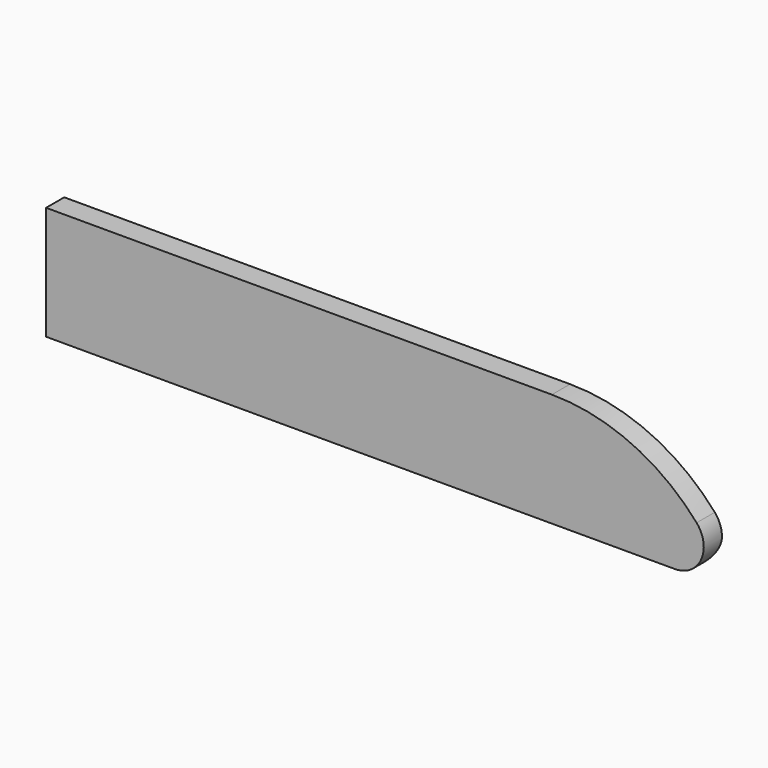
from build123d import *

# Parameters (mm, degrees)
F0_W        = 900
F0_H        = 150
F1_DEPTH    = 30
F2_T1_DEPTH = 1188.6630226256
F3_T1_DEPTH = 405.2304260538
F3_T3_DEPTH = 1086.1451046899


# Not quite as in the source:
# - a fillet or chamfer that OpenCascade refuses, or shapes differently, is made with other operations: its cross-section is extruded or revolved along the edge and cut away or added


with BuildPart() as f1:
    # F0 (on Front) → F1 (new body)
    with BuildSketch(Plane.XZ):
        with Locations((-450, -75)):
            Rectangle(F0_W, F0_H)
    extrude(amount=F1_DEPTH)

    # F2: fillet of radius 254 on 1 edges, made by hand

    # F2_s2 → F2_t1 (cut)
    with BuildSketch(Plane.XZ.offset(-579.3315113128)):
        with BuildLine():
            ThreePointArc((0, -150), (-93.7108671067, -40.7724220463), (-231.7326045251, 0))
            Line((-231.7326045251, 0), (0, 0))
            Line((0, 0), (0, -150))
        make_face()
    extrude(amount=F2_T1_DEPTH, mode=Mode.SUBTRACT)

    # F3: fillet of radius 38.1 on 2 edges, made by hand

    # F3_s2 → F3_t1 (cut)
    with BuildSketch(Plane.XZ.offset(-187.6152130269)):
        with BuildLine():
            ThreePointArc((-69.1890718946, -150), (-34.4974048158, -127.6511344129), (-40.5049190775, -86.8235294118))
            ThreePointArc((-40.5049190775, -86.8235294118), (-17.9063471748, -116.9075798319), (0, -150))
            Line((0, -150), (-69.1890718946, -150))
        make_face()
    extrude(amount=F3_T1_DEPTH, mode=Mode.SUBTRACT)

    # F3_s4 → F3_t3 (cut)
    with BuildSketch(Plane.YZ.offset(-993.0725523449)):
        with BuildLine():
            ThreePointArc((-30, -150), (-8.4333520599, -136.6770452378), (0, -112.770979062))
            Line((0, -112.770979062), (0, -150))
            Line((0, -150), (-30, -150))
        make_face()
    extrude(amount=F3_T3_DEPTH, mode=Mode.SUBTRACT)


solid = f1.part
